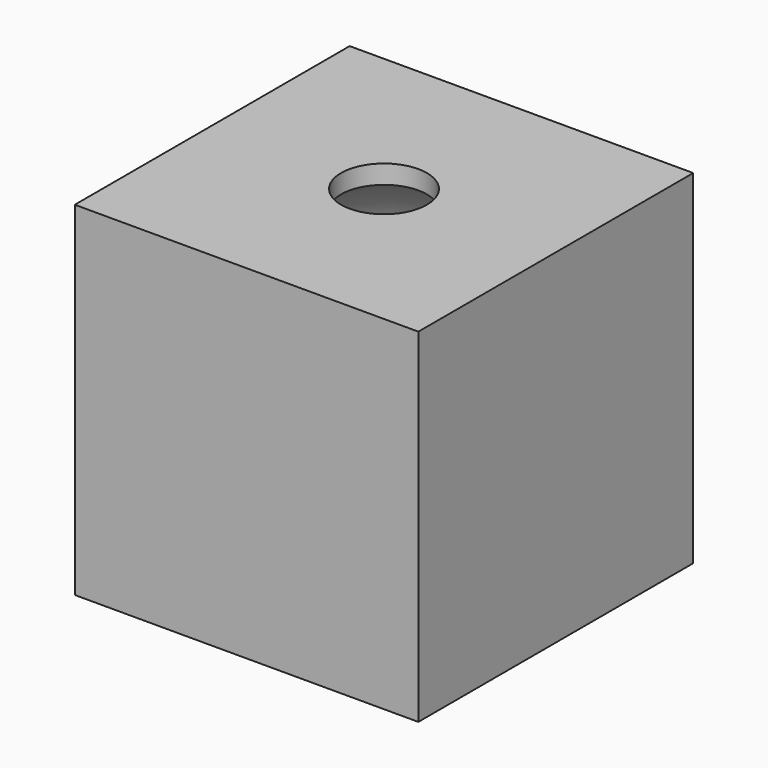
from build123d import *

# Parameters (mm, degrees)
F2_W          = 80
F2_H          = 80
F3_DEPTH      = 40
F7_ANGLE_BACK = 35
F7_ANGLE      = 70
F8_R          = 3
F9_DEPTH      = 4
F10_R         = 10
F11_DEPTH     = 5
F12_R         = 10
F13_DEPTH     = 5


# Not quite as in the source:
# - a feature names something its author has since deleted; it is built from what else it names


with BuildPart() as f1:
    # F0 (on Top) → F1 (revolve)
    with BuildSketch(Plane.XY):
        with BuildLine():
            Line((0, 37), (0, -37))
            ThreePointArc((0, -37), (37, 0), (0, 37))
        make_face()
    revolve(axis=Axis((0, 0, 0), (0, -1, 0)))


with BuildPart() as f3:
    # F2 (on Top) → F3 (new body, symmetric)
    with BuildSketch(Plane.XY):
        Rectangle(F2_W, F2_H)
    extrude(amount=F3_DEPTH, both=True)

    # F4: cut F1
    add(f1.part, mode=Mode.SUBTRACT)

    # F6 (on Front) → F7 (revolve)
    with BuildSketch(Plane.XZ, mode=Mode.PRIVATE) as f7_sk:
        with BuildLine():
            add(Edge.make_bspline(
                [(-28.4972605327, -23.5988589159), (-22.613415631, -15.226576282), (-15.2284997687, -1.2521191935), (-21.0733372873, 17.730814669), (-28.4972605327, 23.5988589159)],
                knots=[0, 0, 0, 0, 0.5, 1, 1, 1, 1], degree=3))
            ThreePointArc((-28.4972605327, 23.5988589159), (-29.0776083413, 22.8799626999), (-29.6398253299, 22.1468000942))
            add(Edge.make_bspline(
                [(-29.6398253299, 22.1468000942), (-23.6962903291, 15.970768407), (-17.3082405815, -0.7806496907), (-24.5547182858, -14.3142519519), (-29.8117857382, -21.9147765469)],
                knots=[0, 0, 0, 0, 0.5007860737, 1, 1, 1, 1], degree=3))
            ThreePointArc((-29.8117857382, -21.9147765469), (-29.1666805209, -22.7663072849), (-28.4972605327, -23.5988589159))
        make_face()
    revolve(f7_sk.sketch.rotate(Axis((-40, 0, 0), (0, 0, -1)), -F7_ANGLE_BACK), axis=Axis((-40, 0, 0), (0, 0, -1)), revolution_arc=F7_ANGLE)

    # F8 (on face) → F9 (cut, symmetric)
    with BuildSketch(Plane(origin=(-40, 0, 0), x_dir=(0, -1, 0), z_dir=(-1, 0, 0))):
        Circle(F8_R)
    extrude(amount=F9_DEPTH, both=True, mode=Mode.SUBTRACT)

    # F10 (on face) → F11 (cut, symmetric)
    with BuildSketch(Plane.XY.offset(40)):
        Circle(F10_R)
    extrude(amount=F11_DEPTH, both=True, mode=Mode.SUBTRACT)

    # F12 (on face) → F13 (cut, symmetric)
    with BuildSketch(Plane(origin=(0, 0, -40), x_dir=(1, 0, 0), z_dir=(0, 0, -1))):
        Circle(F12_R)
    extrude(amount=F13_DEPTH, both=True, mode=Mode.SUBTRACT)


solid = f3.part
